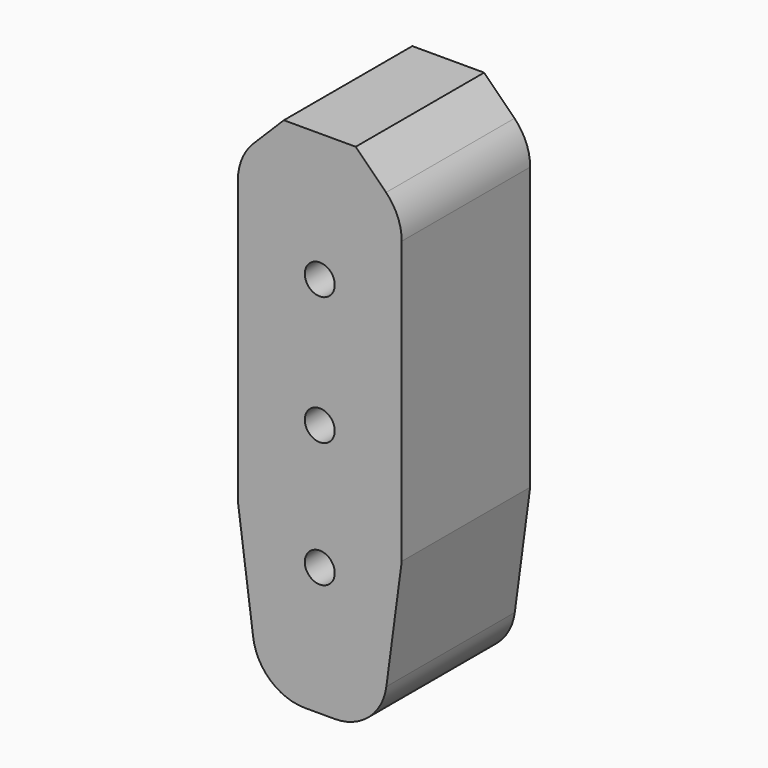
from build123d import *

# Parameters (mm, degrees)
F0_W       = 38.89502
F0_H       = 121.158
F1_DEPTH   = 38.1
F2_SIZE    = 10.922
F3_R       = 12.7
F4_SIZE2   = 5.08
F4_SIZE    = 38.1
F4_2_SIZE2 = 5.08
F4_2_SIZE  = 38.1
F5_R       = 12.3825
F6_R       = 5.08
F6_R_2     = 3.556
F7_DEPTH   = 12.7
F8_DEPTH   = 38.101


with BuildPart() as f1:
    # F0 (on Front) → F1 (new body)
    with BuildSketch(Plane.XZ):
        with Locations((0, -9.779)):
            Rectangle(F0_W, F0_H)
    extrude(amount=-F1_DEPTH)

    # F2
    f2_edges = [f1.edges().sort_by_distance(p)[0] for p in [
        (19.44751, 19.05, 50.8),
        (-19.44751, 19.05, 50.8),
    ]]
    chamfer(f2_edges, length=F2_SIZE)

    # F3
    f3_edges = [f1.edges().sort_by_distance(p)[0] for p in [
        (19.44751, 19.05, 39.878),
        (-19.44751, 19.05, 39.878),
    ]]
    fillet(f3_edges, radius=F3_R)

    # F4
    f4_edges = [f1.edges().sort_by_distance(p)[0] for p in [
        (-19.44751, 19.05, -70.358),
    ]]
    f4_side = f1.faces().sort_by_distance((-19.44751, 19.05, -17.870256))[0]
    chamfer(f4_edges, length=F4_SIZE, length2=F4_SIZE2, reference=f4_side)

    # F4#2
    f4_2_edges = [f1.edges().sort_by_distance(p)[0] for p in [
        (19.44751, 19.05, -70.358),
    ]]
    f4_2_side = f1.faces().sort_by_distance((19.44751, 19.05, -17.870256))[0]
    chamfer(f4_2_edges, length=F4_2_SIZE, length2=F4_2_SIZE2, reference=f4_2_side)

    # F5
    f5_edges = [f1.edges().sort_by_distance(p)[0] for p in [
        (14.36751, 19.05, -70.358),
        (-14.36751, 19.05, -70.358),
    ]]
    fillet(f5_edges, radius=F5_R)

    # F6 (on face) → F7 (cut)
    with BuildSketch(Plane(origin=(0, 38.1, 0), x_dir=(-1, 0, 0), z_dir=(0, 1, 0))):
        with Locations((0, -39.878)):
            Circle(F6_R)
        with Locations((0, -39.878)):
            Circle(F6_R_2, mode=Mode.SUBTRACT)
        with Locations((0, -10.16)):
            Circle(F6_R)
        with Locations((0, -10.16)):
            Circle(F6_R_2, mode=Mode.SUBTRACT)
        with Locations((0, 20.32)):
            Circle(F6_R)
        with Locations((0, 20.32)):
            Circle(F6_R_2, mode=Mode.SUBTRACT)
    extrude(amount=-F7_DEPTH, mode=Mode.SUBTRACT)

    # F6 (on face) → F8 (cut, through all)
    with BuildSketch(Plane(origin=(0, 38.1, 0), x_dir=(-1, 0, 0), z_dir=(0, 1, 0))):
        with Locations((0, 20.32)):
            Circle(F6_R_2)
        with Locations((0, -10.16)):
            Circle(F6_R_2)
        with Locations((0, -39.878)):
            Circle(F6_R_2)
    extrude(amount=-F8_DEPTH, mode=Mode.SUBTRACT)


solid = f1.part
